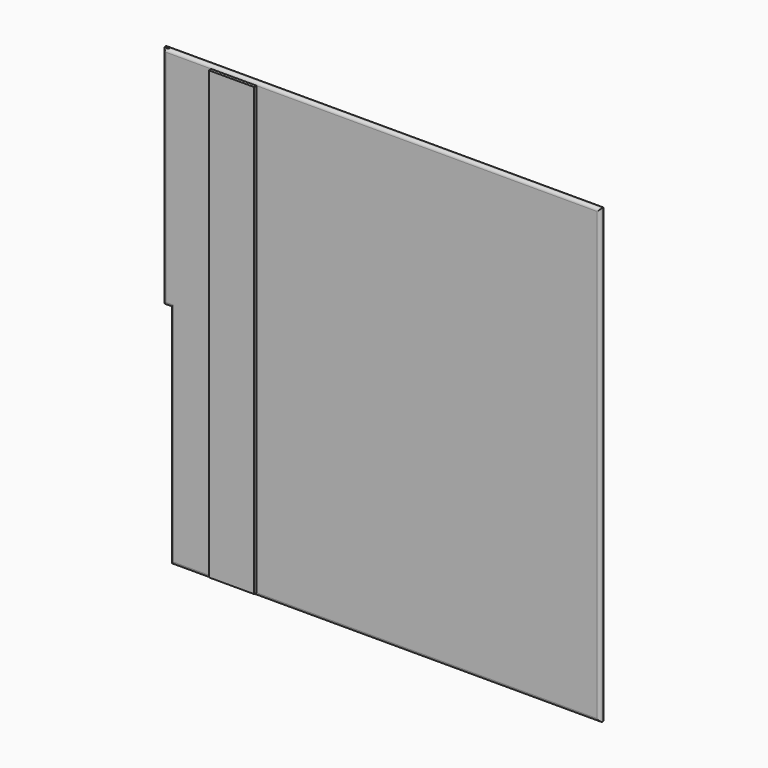
from build123d import *

# Parameters (mm, degrees)
F1_DEPTH     = 4
F2_R         = 1
F3_DEPTH     = 310
F4_T1_DEPTH  = 300
F4_T3_DEPTH  = 160
F4_T5_DEPTH  = 10
F4_T7_DEPTH  = 155
F4_T9_DEPTH  = 295
F4_T11_DEPTH = 310
F4_T17_DEPTH = 15
F4_T21_DEPTH = 160
F5_T1_DEPTH  = 300
F5_T3_DEPTH  = 160
F5_T5_DEPTH  = 10
F5_T7_DEPTH  = 155
F5_T9_DEPTH  = 295
F5_T11_DEPTH = 310
F5_T17_DEPTH = 15
F5_T21_DEPTH = 160
F6_W         = 30
F6_H         = 296
F7_DEPTH     = 2


# Not quite as in the source:
# - a fillet or chamfer that OpenCascade refuses, or shapes differently, is made with other operations: its cross-section is extruded or revolved along the edge and cut away or added


with BuildPart() as f1:
    # F0 (on Front) → F1 (new body)
    with BuildSketch(Plane.XZ):
        Polygon((251.4121359825, 250.8489221025), (-38.5878640175, 250.8489221025), (-38.5878640175, 100.8489221025), (-33.5878640175, 100.8489221025), (-33.5878640175, -49.1510778975), (251.4121359825, -49.1510778975), align=None)
    extrude(amount=F1_DEPTH)

    # F2 (on face) → F3 (cut)
    with BuildSketch(Plane.XY.offset(250.8489221025)):
        with Locations((-36.5878640175, -2)):
            Circle(F2_R)
    extrude(amount=-F3_DEPTH, mode=Mode.SUBTRACT)

    # F4: fillet of radius 2 on 6 edges, made by hand

    # F4_s2 → F4_t1 (cut)
    with BuildSketch(Plane.YZ.offset(-43.5878640175)):
        with BuildLine():
            ThreePointArc((-2, 250.8489221025), (-3.4142135624, 250.2631356648), (-4, 248.8489221025))
            Line((-4, 248.8489221025), (-4, 250.8489221025))
            Line((-4, 250.8489221025), (-2, 250.8489221025))
        make_face()
    extrude(amount=F4_T1_DEPTH, mode=Mode.SUBTRACT)

    # F4_s4 → F4_t3 (cut)
    with BuildSketch(Plane.XY.offset(95.8489221025)):
        with BuildLine():
            ThreePointArc((-36.5878640175, -4), (-38.0020775799, -3.4142135624), (-38.5878640175, -2))
            Line((-38.5878640175, -2), (-38.5878640175, -4))
            Line((-38.5878640175, -4), (-36.5878640175, -4))
        make_face()
    extrude(amount=F4_T3_DEPTH, mode=Mode.SUBTRACT)

    # F4_s6 → F4_t5 (cut)
    with BuildSketch(Plane.YZ.offset(-43.5878640175)):
        with BuildLine():
            ThreePointArc((-4, 102.8489221025), (-3.4142135624, 101.4347085401), (-2, 100.8489221025))
            Line((-2, 100.8489221025), (-4, 100.8489221025))
            Line((-4, 100.8489221025), (-4, 102.8489221025))
        make_face()
    extrude(amount=F4_T5_DEPTH, mode=Mode.SUBTRACT)

    # F4_s8 → F4_t7 (cut)
    with BuildSketch(Plane.XY.offset(-54.1510778975)):
        with BuildLine():
            ThreePointArc((-31.5878640175, -4), (-33.0020775799, -3.4142135624), (-33.5878640175, -2))
            Line((-33.5878640175, -2), (-33.5878640175, -4))
            Line((-33.5878640175, -4), (-31.5878640175, -4))
        make_face()
    extrude(amount=F4_T7_DEPTH, mode=Mode.SUBTRACT)

    # F4_s10 → F4_t9 (cut)
    with BuildSketch(Plane.YZ.offset(-38.5878640175)):
        with BuildLine():
            ThreePointArc((-4, -47.1510778975), (-3.4142135624, -48.5652914599), (-2, -49.1510778975))
            Line((-2, -49.1510778975), (-4, -49.1510778975))
            Line((-4, -49.1510778975), (-4, -47.1510778975))
        make_face()
    extrude(amount=F4_T9_DEPTH, mode=Mode.SUBTRACT)

    # F4_s12 → F4_t11 (cut)
    with BuildSketch(Plane.XY.offset(-54.1510778975)):
        with BuildLine():
            ThreePointArc((251.4121359825, -2), (250.8263495449, -3.4142135624), (249.4121359825, -4))
            Line((249.4121359825, -4), (251.4121359825, -4))
            Line((251.4121359825, -4), (251.4121359825, -2))
        make_face()
    extrude(amount=F4_T11_DEPTH, mode=Mode.SUBTRACT)


with BuildPart() as f4_tool15:
    # F4_s16 → F4_t17 (new body)
    with BuildSketch(Plane.YZ.offset(-43.5878640175)):
        with BuildLine():
            ThreePointArc((-4, 102.8489221025), (-3.4142135624, 101.4347085401), (-2, 100.8489221025))
            Line((-2, 100.8489221025), (-4, 100.8489221025))
            Line((-4, 100.8489221025), (-4, 102.8489221025))
        make_face()
    extrude(amount=F4_T17_DEPTH)

    split(bisect_by=Plane.YZ.offset(-33.5878640175), keep=Keep.TOP)


with BuildPart() as f4_tool19:
    # F4_s20 → F4_t21 (new body)
    with BuildSketch(Plane.XY.offset(105.8489221025)):
        with BuildLine():
            ThreePointArc((-31.5878640175, -4), (-33.0020775799, -3.4142135624), (-33.5878640175, -2))
            Line((-33.5878640175, -2), (-33.5878640175, -4))
            Line((-33.5878640175, -4), (-31.5878640175, -4))
        make_face()
    extrude(amount=-F4_T21_DEPTH)

    split(bisect_by=Plane.XY.offset(100.8489221025), keep=Keep.TOP)


with BuildPart() as f4_tool15_1:
    add(f4_tool15.part)

    # F4_t23: intersect F4_tool19
    add(f4_tool19.part, mode=Mode.INTERSECT)


with BuildPart() as f1_1:
    add(f1.part)

    # F4_t13: cut F4_tool15
    add(f4_tool15_1.part, mode=Mode.SUBTRACT)

    # F5: fillet of radius 2 on 6 edges, made by hand

    # F5_s2 → F5_t1 (cut)
    with BuildSketch(Plane.YZ.offset(-43.5878640175)):
        with BuildLine():
            ThreePointArc((-2, 250.8489221025), (-0.5857864376, 250.2631356648), (0, 248.8489221025))
            Line((0, 248.8489221025), (0, 250.8489221025))
            Line((0, 250.8489221025), (-2, 250.8489221025))
        make_face()
    extrude(amount=F5_T1_DEPTH, mode=Mode.SUBTRACT)

    # F5_s4 → F5_t3 (cut)
    with BuildSketch(Plane.XY.offset(95.8489221025)):
        with BuildLine():
            ThreePointArc((-36.5878640175, 0), (-38.0020775799, -0.5857864376), (-38.5878640175, -2))
            Line((-38.5878640175, -2), (-38.5878640175, 0))
            Line((-38.5878640175, 0), (-36.5878640175, 0))
        make_face()
    extrude(amount=F5_T3_DEPTH, mode=Mode.SUBTRACT)

    # F5_s6 → F5_t5 (cut)
    with BuildSketch(Plane.YZ.offset(-43.5878640175)):
        with BuildLine():
            ThreePointArc((0, 102.8489221025), (-0.5857864376, 101.4347085401), (-2, 100.8489221025))
            Line((-2, 100.8489221025), (0, 100.8489221025))
            Line((0, 100.8489221025), (0, 102.8489221025))
        make_face()
    extrude(amount=F5_T5_DEPTH, mode=Mode.SUBTRACT)

    # F5_s8 → F5_t7 (cut)
    with BuildSketch(Plane.XY.offset(-54.1510778975)):
        with BuildLine():
            ThreePointArc((-31.5878640175, 0), (-33.0020775799, -0.5857864376), (-33.5878640175, -2))
            Line((-33.5878640175, -2), (-33.5878640175, 0))
            Line((-33.5878640175, 0), (-31.5878640175, 0))
        make_face()
    extrude(amount=F5_T7_DEPTH, mode=Mode.SUBTRACT)

    # F5_s10 → F5_t9 (cut)
    with BuildSketch(Plane.YZ.offset(-38.5878640175)):
        with BuildLine():
            ThreePointArc((0, -47.1510778975), (-0.5857864376, -48.5652914599), (-2, -49.1510778975))
            Line((-2, -49.1510778975), (0, -49.1510778975))
            Line((0, -49.1510778975), (0, -47.1510778975))
        make_face()
    extrude(amount=F5_T9_DEPTH, mode=Mode.SUBTRACT)

    # F5_s12 → F5_t11 (cut)
    with BuildSketch(Plane.XY.offset(-54.1510778975)):
        with BuildLine():
            ThreePointArc((249.4121359825, 0), (250.8263495449, -0.5857864376), (251.4121359825, -2))
            Line((251.4121359825, -2), (251.4121359825, 0))
            Line((251.4121359825, 0), (249.4121359825, 0))
        make_face()
    extrude(amount=F5_T11_DEPTH, mode=Mode.SUBTRACT)


with BuildPart() as f5_tool15:
    # F5_s16 → F5_t17 (new body)
    with BuildSketch(Plane.YZ.offset(-43.5878640175)):
        with BuildLine():
            ThreePointArc((0, 102.8489221025), (-0.5857864376, 101.4347085401), (-2, 100.8489221025))
            Line((-2, 100.8489221025), (0, 100.8489221025))
            Line((0, 100.8489221025), (0, 102.8489221025))
        make_face()
    extrude(amount=F5_T17_DEPTH)

    split(bisect_by=Plane.YZ.offset(-33.5878640175), keep=Keep.TOP)


with BuildPart() as f5_tool19:
    # F5_s20 → F5_t21 (new body)
    with BuildSketch(Plane.XY.offset(105.8489221025)):
        with BuildLine():
            ThreePointArc((-31.5878640175, 0), (-33.0020775799, -0.5857864376), (-33.5878640175, -2))
            Line((-33.5878640175, -2), (-33.5878640175, 0))
            Line((-33.5878640175, 0), (-31.5878640175, 0))
        make_face()
    extrude(amount=-F5_T21_DEPTH)

    split(bisect_by=Plane.XY.offset(100.8489221025), keep=Keep.TOP)


with BuildPart() as f5_tool15_1:
    add(f5_tool15.part)

    # F5_t23: intersect F5_tool19
    add(f5_tool19.part, mode=Mode.INTERSECT)


with BuildPart() as f1_2:
    add(f1_1.part)

    # F5_t13: cut F5_tool15
    add(f5_tool15_1.part, mode=Mode.SUBTRACT)

    # F6 (on face) → F7 (join)
    with BuildSketch(Plane.XZ.offset(4)):
        with Locations((8.4121359825, 100.8489221025)):
            Rectangle(F6_W, F6_H)
    extrude(amount=F7_DEPTH)


solid = f1_2.part
